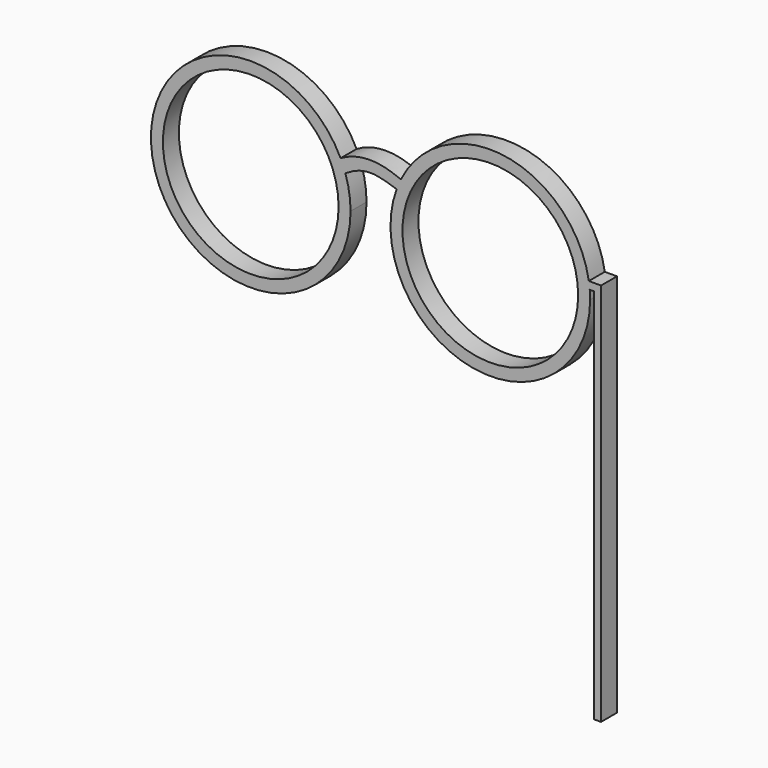
from build123d import *

# Parameters (mm, degrees)
F0_R     = 4.4
F1_DEPTH = 1


with BuildPart() as f1:
    # F0 (on Front) → F1 (new body)
    with BuildSketch(Plane.XZ):
        with BuildLine():
            ThreePointArc((-1.4986815922, 5.1042757445), (-10.8737353251, 1.8109915545), (-1, 2.9275505456))
            ThreePointArc((-1, 2.9275505456), (-1.0654410934, 3.733855945), (-1.2600513589, 4.5190551417))
            ThreePointArc((-1.2600513589, 4.5190551417), (-1.3701106972, 4.81543959), (-1.4986815922, 5.1042757445))
        make_face()
        with Locations((-6, 2.9275505456)):
            Circle(F0_R, mode=Mode.SUBTRACT)
        with BuildLine():
            ThreePointArc((-1.4986815922, 5.1042757445), (-1.3701106972, 4.81543959), (-1.2600513589, 4.5190551417))
            add(Edge.make_bspline(
                [(-1.2600513589, 4.5190551417), (-0.3321453987, 5.1084347069), (0.2222434123, 5.0197322853), (1.305815297, 4.6493606322)],
                knots=[0, 0, 0, 0, 2.5691732555, 2.5691732555, 2.5691732555, 2.5691732555], degree=3))
            ThreePointArc((1.305815297, 4.6493606322), (1.408443121, 4.9068447194), (1.525181814, 5.1582459982))
            add(Edge.make_bspline(
                [(-1.4986815922, 5.1042757445), (0, 5.9878164902), (1.4394625627, 5.1295237069), (1.525181814, 5.1582459982)],
                knots=[0, 0, 0, 0, 0.9403135209, 0.9403135209, 0.9403135209, 0.9403135209], degree=3))
        make_face()
        with BuildLine():
            ThreePointArc((1.525181814, 5.1582459982), (1.408443121, 4.9068447194), (1.305815297, 4.6493606322))
            ThreePointArc((1.305815297, 4.6493606322), (5.1256212248, -1.9954019991), (11, 2.9275505456))
            ThreePointArc((11, 2.9275505456), (10.9952473554, 3.1455043436), (10.9809984568, 3.3630437989))
            ThreePointArc((10.9809984568, 3.3630437989), (10.9614239437, 3.5474476752), (10.9350249024, 3.7309988718))
            ThreePointArc((10.9350249024, 3.7309988718), (6.7558272917, 7.8700929182), (1.5306314581, 5.1691448079))
            add(Edge.make_bspline(
                [(1.525181814, 5.1582459982), (1.5306228506, 5.160069148), (1.5306095387, 5.165466158), (1.5306314581, 5.1691448079)],
                knots=[0.9403135209, 0.9403135209, 0.9403135209, 0.9403135209, 1, 1, 1, 1], degree=3))
        make_face()
        with Locations((6, 2.9275505456)):
            Circle(F0_R, mode=Mode.SUBTRACT)
        with BuildLine():
            ThreePointArc((10.9350249024, 3.7309988718), (10.9614239437, 3.5474476752), (10.9809984568, 3.3630437989))
            Line((10.9809984568, 3.3630437989), (11.1943203956, 3.3630437989))
            Line((11.1943203956, 3.3630437989), (11.1943203956, -15.5131826177))
            Line((11.1943203956, -15.5131826177), (11.5463633525, -15.5131826177))
            Line((11.5463633525, -15.5131826177), (11.5463633525, 3.7309988718))
            Line((11.5463633525, 3.7309988718), (10.9350249024, 3.7309988718))
        make_face()
    extrude(amount=F1_DEPTH)


solid = f1.part
